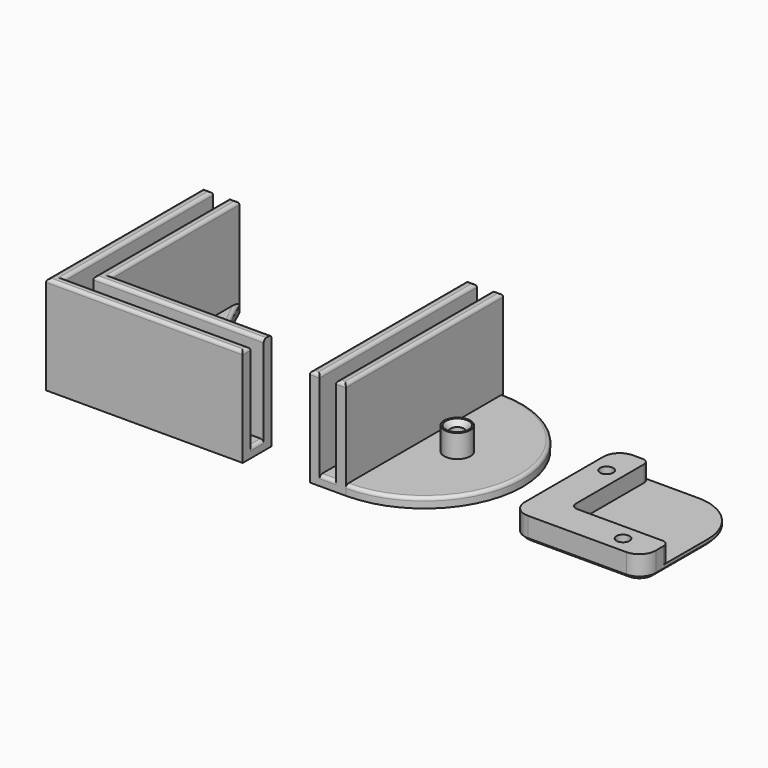
from build123d import *

# Parameters (mm, degrees)
F0_R      = 4
F1_DEPTH  = 3
F2_DEPTH  = 30
F0_R_2    = 2
F3_DEPTH  = 10
F4_R      = 1
F5_SIZE   = 1.5
F6_W      = 5
F6_H      = 60
F7_DEPTH  = 3
F6_R      = 4
F6_W_2    = 3
F8_DEPTH  = 30
F6_R_2    = 2
F9_DEPTH  = 10
F10_SIZE  = 1.5
F11_R     = 1
F12_W     = 40
F12_H     = 40
F13_DEPTH = 7
F14_W     = 30
F14_H     = 30
F15_DEPTH = 5
F14_R     = 2
F16_DEPTH = 25
F17_R     = 3
F17_R_2   = 2
F18_DEPTH = 3
F19_R     = 15
F20_R     = 5
F21_SIZE  = 0.99999
F22_R     = 2


# Not quite as in the source:
# - a fillet or chamfer is up to 0.001 mm smaller than in the source, because OpenCascade refuses the exact size


with BuildPart() as f1:
    # F0 (on Top) → F1 (new body)
    with BuildSketch(Plane.XY):
        with BuildLine():
            ThreePointArc((-18.7818011097, -19.7000644691), (-48.186838974, -0.1051023334), (-67.7818011097, 29.2999355309))
            Line((-67.7818011097, 29.2999355309), (-67.7818011097, -19.7000644691))
            Line((-67.7818011097, -19.7000644691), (-18.7818011097, -19.7000644691))
        make_face()
        with Locations((-57.7818011097, -9.7000644691)):
            Circle(F0_R, mode=Mode.SUBTRACT)
    extrude(amount=F1_DEPTH)



with BuildPart() as f1b:
    # F0 (on Top) → F1, piece 2 (new body)
    with BuildSketch(Plane.XY):
        Polygon((-70.7818011097, 29.2999355309), (-75.7818011097, 29.2999355309), (-75.7818011097, -27.7000644691), (-18.7818011097, -27.7000644691), (-18.7818011097, -22.7000644691), (-70.7818011097, -22.7000644691), align=None)
    extrude(amount=F1_DEPTH)


with BuildPart() as f1_1:
    add(f1.part)

    add(f1b.part)  # F2 merges F1b
    # F0 (on Top) → F2 (join)
    with BuildSketch(Plane.XY):
        Polygon((-75.7818011097, 29.2999355309), (-78.7818011097, 29.2999355309), (-78.7818011097, -30.7000644691), (-18.7818011097, -30.7000644691), (-18.7818011097, -27.7000644691), (-75.7818011097, -27.7000644691), align=None)
        Polygon((-67.7818011097, 29.2999355309), (-70.7818011097, 29.2999355309), (-70.7818011097, -22.7000644691), (-18.7818011097, -22.7000644691), (-18.7818011097, -19.7000644691), (-67.7818011097, -19.7000644691), align=None)
    extrude(amount=F2_DEPTH)

    # F0 (on Top) → F3 (join)
    with BuildSketch(Plane.XY):
        with Locations((-57.7818011097, -9.7000644691)):
            Circle(F0_R)
        with Locations((-57.7818011097, -9.7000644691)):
            Circle(F0_R_2, mode=Mode.SUBTRACT)
    extrude(amount=F3_DEPTH)

    # F4
    f4_edges = [f1_1.edges().sort_by_distance(p)[0] for p in [
        (-78.781801, -0.700064, 30),
        (-48.781801, -30.700064, 30),
        (-44.781801, -22.700064, 30),
        (-70.781801, 3.299936, 30),
        (-67.781801, 4.799936, 30),
        (-43.281801, -19.700064, 30),
        (-75.781801, 0.799936, 30),
        (-47.281801, -27.700064, 30),
        (-77.281801, 29.299936, 30),
        (-69.281801, 29.299936, 30),
        (-18.781801, -29.200064, 30),
        (-48.186839, -0.105102, 3),
        (-18.781801, -25.200064, 3),
        (-73.281801, 29.299936, 3),
    ]]
    fillet(f4_edges, radius=F4_R)

    # F5
    f5_edges = [f1_1.edges().sort_by_distance(p)[0] for p in [
        (-59.781801, -9.700064, 10),
    ]]
    chamfer(f5_edges, length=F5_SIZE)


with BuildPart() as f7:
    # F6 (on Top) → F7 (new body)
    with BuildSketch(Plane.XY):
        with Locations((5.5, 1.4149925858)):
            Rectangle(F6_W, F6_H)
    extrude(amount=F7_DEPTH)



with BuildPart() as f7b:
    # F6 (on Top) → F7, piece 2 (new body)
    with BuildSketch(Plane.XY):
        with BuildLine():
            ThreePointArc((11, -28.5850074142), (41, 1.4149925858), (11, 31.4149925858))
            Line((11, 31.4149925858), (11, -28.5850074142))
        make_face()
        with Locations((21, 1.4149925858)):
            Circle(F6_R, mode=Mode.SUBTRACT)
    extrude(amount=F7_DEPTH)


with BuildPart() as f7_1:
    add(f7.part)

    add(f7b.part)  # F8 merges F7b
    # F6 (on Top) → F8 (join)
    with BuildSketch(Plane.XY):
        with Locations((1.5, 1.4149925858)):
            Rectangle(F6_W_2, F6_H)
        with Locations((9.5, 1.4149925858)):
            Rectangle(F6_W_2, F6_H)
    extrude(amount=F8_DEPTH)

    # F6 (on Top) → F9 (join)
    with BuildSketch(Plane.XY):
        with Locations((21, 1.4149925858)):
            Circle(F6_R)
        with Locations((21, 1.4149925858)):
            Circle(F6_R_2, mode=Mode.SUBTRACT)
    extrude(amount=F9_DEPTH)

    # F10
    f10_edges = [f7_1.edges().sort_by_distance(p)[0] for p in [
        (19, 1.414993, 10),
    ]]
    chamfer(f10_edges, length=F10_SIZE)

    # F11
    f11_edges = [f7_1.edges().sort_by_distance(p)[0] for p in [
        (0, 1.414993, 30),
        (3, 1.414993, 30),
        (8, 1.414993, 30),
        (11, 1.414993, 30),
        (9.5, -28.585007, 30),
        (1.5, -28.585007, 30),
        (5.5, -28.585007, 3),
        (41, 1.414993, 3),
        (1.5, 31.414993, 30),
        (9.5, 31.414993, 30),
        (5.5, 31.414993, 3),
    ]]
    fillet(f11_edges, radius=F11_R)


with BuildPart() as f13:
    # F12 (on Top) → F13 (new body)
    with BuildSketch(Plane.XY):
        with Locations((74.6976004541, 0)):
            Rectangle(F12_W, F12_H)
    extrude(amount=F13_DEPTH)

    # F14 (on face) → F15 (cut)
    with BuildSketch(Plane.XY.offset(7)):
        with Locations((79.6976004541, 5)):
            Rectangle(F14_W, F14_H)
    extrude(amount=-F15_DEPTH, mode=Mode.SUBTRACT)

    # F14 (on face) → F16 (cut)
    with BuildSketch(Plane.XY.offset(7)):
        with Locations((59.6976004541, 10)):
            Circle(F14_R)
        with Locations((84.6976004541, -15)):
            Circle(F14_R)
    extrude(amount=-F16_DEPTH, mode=Mode.SUBTRACT)

    # F17 (on face) → F18 (cut)
    with BuildSketch(Plane(origin=(0, 0, 0), x_dir=(1, 0, 0), z_dir=(0, 0, -1))):
        with Locations((59.6976004541, -10)):
            Circle(F17_R)
        with Locations((59.6976004541, -10)):
            Circle(F17_R_2, mode=Mode.SUBTRACT)
        with Locations((84.6976004541, 15)):
            Circle(F17_R)
        with Locations((84.6976004541, 15)):
            Circle(F17_R_2, mode=Mode.SUBTRACT)
    extrude(amount=-F18_DEPTH, mode=Mode.SUBTRACT)

    # F19
    f19_edges = [f13.edges().sort_by_distance(p)[0] for p in [
        (94.6976, 20, 1),
    ]]
    fillet(f19_edges, radius=F19_R)

    # F20
    f20_edges = [f13.edges().sort_by_distance(p)[0] for p in [
        (54.6976, 20, 3.5),
        (94.6976, -20, 3.5),
        (54.6976, -20, 3.5),
    ]]
    fillet(f20_edges, radius=F20_R)

    # F21 (size 1 in the source; OpenCascade refuses exactly that, so slightly less here)
    f21_edges = [f13.edges().sort_by_distance(p)[0] for p in [
        (94.6976, -5, 0),
        (56.6976, 10, 0),
        (81.6976, -15, 0),
    ]]
    chamfer(f21_edges, length=F21_SIZE)

    # F22
    f22_edges = [f13.edges().sort_by_distance(p)[0] for p in [
        (64.6976, 20, 4.5),
        (94.6976, -10, 4.5),
        (64.6976, -10, 4.5),
    ]]
    fillet(f22_edges, radius=F22_R)


solid = Compound([f1_1.part, f7_1.part, f13.part])
